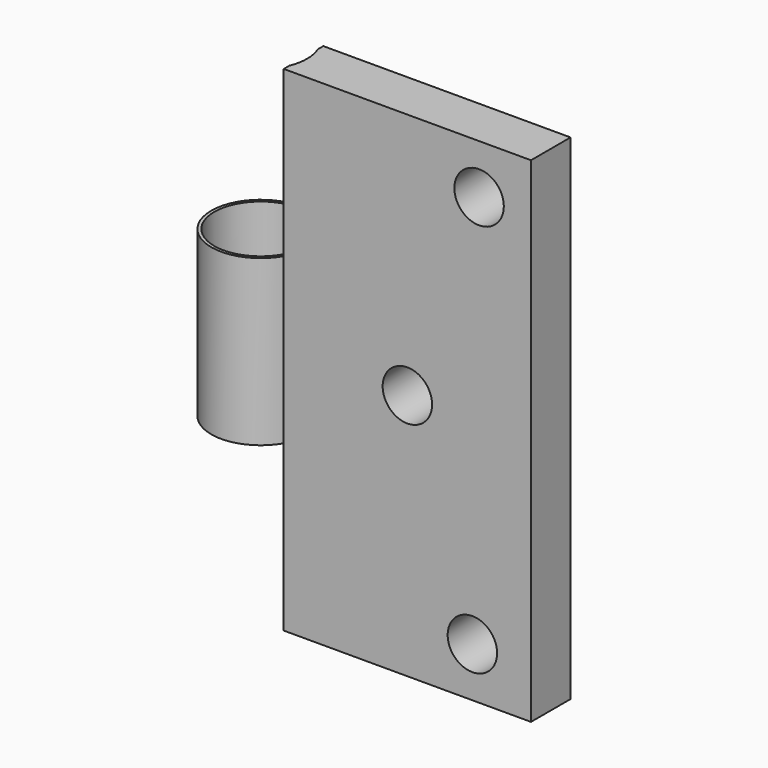
from build123d import *

# Parameters (mm, degrees)
F1_DEPTH      = 127
F2_W          = 29.5337063888
F2_H          = 42.3418
F3_DEPTH      = 25.4
F3_DEPTH_BACK = 25.4
F5_D          = 12.7
F6_D          = 23.8125
F7_ANGLE      = -180


# Not quite as in the source:
# - a length typed as a fraction of an inch, garbled in the dataset ("3 / 203.2 mm" for 3/8 in), is restored


with BuildPart() as f1:
    # F0 (on Top) → F1 (new body)
    with BuildSketch(Plane.XY):
        with BuildLine():
            Line((31.7496773719, 6.35), (-31.75, 6.35))
            Line((-31.75, 6.35), (-31.75, -6.35))
            Line((-31.75, -6.35), (31.7496773719, -6.35))
            ThreePointArc((31.7496773719, -6.35), (30.0482, 0), (31.7496773719, 6.35))
        make_face()
        with BuildLine():
            ThreePointArc((55.4482, 0), (46.0352018728, 12.2672579939), (31.7496773719, 6.35))
            Line((31.7496773719, 6.35), (31.75, 6.35))
            Line((31.75, 6.35), (31.75, -6.35))
            Line((31.75, -6.35), (31.7496773719, -6.35))
            ThreePointArc((31.7496773719, -6.35), (46.0352018728, -12.2672579939), (55.4482, 0))
        make_face()
        with BuildLine():
            Line((31.75, 6.35), (31.7496773719, 6.35))
            ThreePointArc((31.7496773719, 6.35), (30.0482, 0), (31.7496773719, -6.35))
            Line((31.7496773719, -6.35), (31.75, -6.35))
            Line((31.75, -6.35), (31.75, 6.35))
        make_face()
    extrude(amount=-F1_DEPTH)

    # F2 (on face) → F3 (cut, two sides)
    with BuildSketch(Plane.XZ.offset(6.35)) as f3_sk:
        with Locations((46.5165305664, -21.1709)):
            Rectangle(F2_W, F2_H)
        with Locations((46.5165305664, -105.8291)):
            Rectangle(F2_W, F2_H)
    extrude(amount=F3_DEPTH, mode=Mode.SUBTRACT)
    extrude(f3_sk.sketch, amount=-F3_DEPTH_BACK, mode=Mode.SUBTRACT)

    # F5 (through all)
    with Locations(Plane.XZ.offset(6.35)):
        with Locations((-18.4241778449, -12.7), (-16.7022929663, -114.3), (0, -63.5)):
            Hole(F5_D / 2)

    # F6 (through all)
    with Locations(Plane.XY):
        with Locations((42.7482, 0)):
            Hole(F6_D / 2)


with BuildPart() as f1_1:
    # F7: moved
    add(f1.part.rotate(Axis((42.7482, 0, 0), (0, 0, 1)), F7_ANGLE))


solid = f1_1.part
